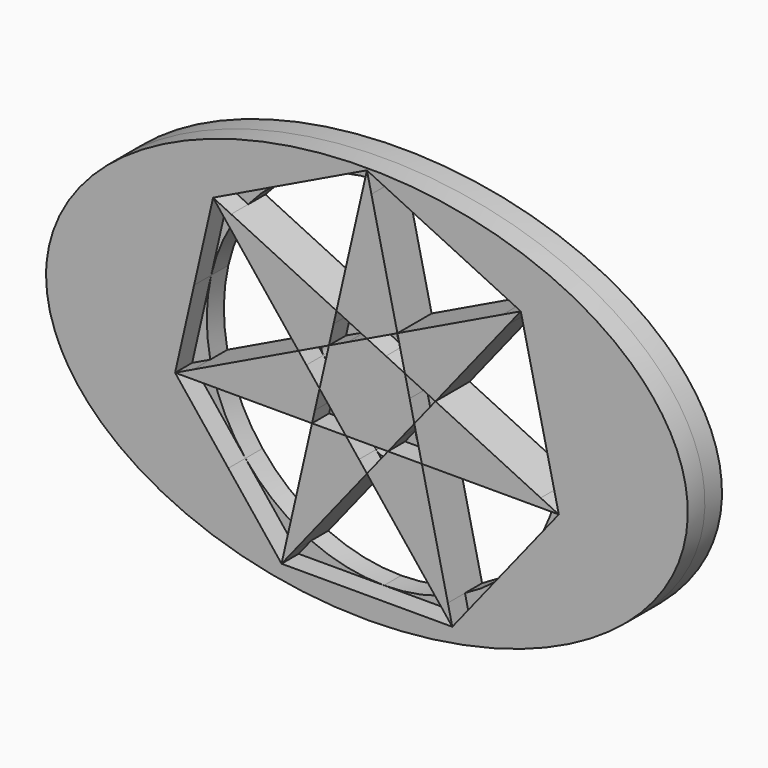
from build123d import *

# Parameters (mm, degrees)
F1_DEPTH = 5
F2_DEPTH = 5


# Not quite as in the source:
# - a feature names something its author has since deleted; it is built from what else it names


with BuildPart() as f1:
    # F0 (on Front) → F1 (new body, symmetric)
    with BuildSketch(Plane.XZ):
        with BuildLine():
            Line((-7.1231604273, 14.7913950385), (-31.742271471, 26.6473340548))
            ThreePointArc((-31.742271471, 26.6473340548), (-32.4026679799, 25.8402654428), (-33.0425496488, 25.0168367919))
            Line((-33.0425496488, 25.0168367919), (-16.0055961941, 3.653172885))
            Line((-16.0055961941, 3.653172885), (-13.3236535657, 4.944728384))
            Line((-13.3236535657, 4.944728384), (-8.8824357668, 7.0835061525))
            Line((-8.8824357668, 7.0835061525), (-7.7855455192, 11.8892963316))
            Line((-7.7855455192, 11.8892963316), (-7.1231604273, 14.7913950385))
        make_face()
        with BuildLine():
            Line((-31.742271471, 26.6473340548), (-35.9642481935, 28.6805308855))
            Line((-35.9642481935, 28.6805308855), (-33.0425496488, 25.0168367919))
            ThreePointArc((-33.0425496488, 25.0168367919), (-32.4026679799, 25.8402654428), (-31.742271471, 26.6473340548))
        make_face()
    extrude(amount=F1_DEPTH, both=True)


with BuildPart() as f1b:
    # F0 (on Front) → F1, piece 2 (new body, symmetric)
    with BuildSketch(Plane.XZ):
        with BuildLine():
            ThreePointArc((-40.6247072379, -8.2027661312), (-40.4054660769, -9.2222839618), (-40.1606433291, -10.235962962))
            Line((-40.1606433291, -10.235962962), (-12.8354915721, -10.235962962))
            Line((-12.8354915721, -10.235962962), (-12.1731064643, -7.3338641855))
            Line((-12.1731064643, -7.3338641855), (-11.0762162326, -2.528074076))
            Line((-11.0762162326, -2.528074076), (-14.1496343689, 1.3258703679))
            Line((-14.1496343689, 1.3258703679), (-16.0055961941, 3.653172885))
            Line((-16.0055961941, 3.653172885), (-40.6247072379, -8.2027661312))
        make_face()
        with BuildLine():
            Line((-40.6247072379, -8.2027661312), (-44.8466839604, -10.235962962))
            Line((-44.8466839604, -10.235962962), (-40.1606433291, -10.235962962))
            ThreePointArc((-40.1606433291, -10.235962962), (-40.4054660769, -9.2222839618), (-40.6247072379, -8.2027661312))
        make_face()
    extrude(amount=F1_DEPTH, both=True)


with BuildPart() as f1c:
    # F0 (on Front) → F1, piece 3 (new body, symmetric)
    with BuildSketch(Plane.XZ):
        with BuildLine():
            ThreePointArc((-18.9159098616, -36.8760161145), (-17.9821240968, -37.3402654428), (-17.0369534547, -37.7808738299))
            Line((-17.0369534547, -37.7808738299), (0, -16.417209923))
            Line((0, -16.417209923), (-1.85596184, -14.0899073875))
            Line((-1.85596184, -14.0899073875), (-4.9293799615, -10.235962962))
            Line((-4.9293799615, -10.235962962), (-9.8587599231, -10.235962962))
            Line((-9.8587599231, -10.235962962), (-12.8354915721, -10.235962962))
            Line((-12.8354915721, -10.235962962), (-18.9159098616, -36.8760161145))
        make_face()
        with BuildLine():
            Line((-18.9159098616, -36.8760161145), (-19.9586519994, -41.4445679235))
            Line((-19.9586519994, -41.4445679235), (-17.0369534547, -37.7808738299))
            ThreePointArc((-17.0369534547, -37.7808738299), (-17.9821240968, -37.3402654428), (-18.9159098616, -36.8760161145))
        make_face()
    extrude(amount=F1_DEPTH, both=True)


with BuildPart() as f1d:
    # F0 (on Front) → F1, piece 4 (new body, symmetric)
    with BuildSketch(Plane.XZ):
        with BuildLine():
            Line((0, -16.417209923), (17.0369534547, -37.7808738299))
            ThreePointArc((17.0369534547, -37.7808738299), (17.9821240968, -37.3402654428), (18.9159098616, -36.8760161145))
            Line((18.9159098616, -36.8760161145), (12.8354915721, -10.235962962))
            Line((12.8354915721, -10.235962962), (9.8587599151, -10.235962962))
            Line((9.8587599151, -10.235962962), (4.9293799615, -10.235962962))
            Line((4.9293799615, -10.235962962), (1.8559618555, -14.089907368))
            Line((1.8559618555, -14.089907368), (0, -16.417209923))
        make_face()
        with BuildLine():
            Line((17.0369534547, -37.7808738299), (19.9586519994, -41.4445679235))
            Line((19.9586519994, -41.4445679235), (18.9159098616, -36.8760161145))
            ThreePointArc((18.9159098616, -36.8760161145), (17.9821240968, -37.3402654428), (17.0369534547, -37.7808738299))
        make_face()
    extrude(amount=F1_DEPTH, both=True)


with BuildPart() as f1e:
    # F0 (on Front) → F1, piece 5 (new body, symmetric)
    with BuildSketch(Plane.XZ):
        with BuildLine():
            ThreePointArc((40.1606433291, -10.235962962), (40.4054660769, -9.2222839618), (40.6247072379, -8.2027661312))
            Line((40.6247072379, -8.2027661312), (16.0055961941, 3.653172885))
            Line((16.0055961941, 3.653172885), (14.1496343961, 1.3258704021))
            Line((14.1496343961, 1.3258704021), (11.0762162326, -2.528074076))
            Line((11.0762162326, -2.528074076), (12.1731064608, -7.3338641702))
            Line((12.1731064608, -7.3338641702), (12.8354915721, -10.235962962))
            Line((12.8354915721, -10.235962962), (40.1606433291, -10.235962962))
        make_face()
        with BuildLine():
            Line((40.1606433291, -10.235962962), (44.8466839604, -10.235962962))
            Line((44.8466839604, -10.235962962), (40.6247072379, -8.2027661312))
            ThreePointArc((40.6247072379, -8.2027661312), (40.4054660769, -9.2222839618), (40.1606433291, -10.235962962))
        make_face()
    extrude(amount=F1_DEPTH, both=True)


with BuildPart() as f1f:
    # F0 (on Front) → F1, piece 6 (new body, symmetric)
    with BuildSketch(Plane.XZ):
        with BuildLine():
            Line((16.0055961941, 3.653172885), (33.0425496488, 25.0168367919))
            ThreePointArc((33.0425496488, 25.0168367919), (32.4026679799, 25.8402654428), (31.742271471, 26.6473340548))
            Line((31.742271471, 26.6473340548), (7.1231604273, 14.7913950385))
            Line((7.1231604273, 14.7913950385), (7.7855455438, 11.8892962237))
            Line((7.7855455438, 11.8892962237), (8.8824357668, 7.0835061525))
            Line((8.8824357668, 7.0835061525), (13.3236536413, 4.9447283476))
            Line((13.3236536413, 4.9447283476), (16.0055961941, 3.653172885))
        make_face()
        with BuildLine():
            Line((33.0425496488, 25.0168367919), (35.9642481935, 28.6805308855))
            Line((35.9642481935, 28.6805308855), (31.742271471, 26.6473340548))
            ThreePointArc((31.742271471, 26.6473340548), (32.4026679799, 25.8402654428), (33.0425496488, 25.0168367919))
        make_face()
    extrude(amount=F1_DEPTH, both=True)


with BuildPart() as f1g:
    # F0 (on Front) → F1, piece 7 (new body, symmetric)
    with BuildSketch(Plane.XZ):
        with BuildLine():
            Line((7.1231604273, 14.7913950385), (1.0427421378, 41.431448191))
            ThreePointArc((1.0427421378, 41.431448191), (0, 41.4445679235), (-1.0427421378, 41.431448191))
            Line((-1.0427421378, 41.431448191), (-7.1231604273, 14.7913950385))
            Line((-7.1231604273, 14.7913950385), (-4.4412178209, 13.4998395501))
            Line((-4.4412178209, 13.4998395501), (0, 11.361061771))
            Line((0, 11.361061771), (4.4412179301, 13.4998396027))
            Line((4.4412179301, 13.4998396027), (7.1231604273, 14.7913950385))
        make_face()
        with BuildLine():
            Line((1.0427421378, 41.431448191), (0, 46))
            Line((0, 46), (-1.0427421378, 41.431448191))
            ThreePointArc((-1.0427421378, 41.431448191), (0, 41.4445679235), (1.0427421378, 41.431448191))
        make_face()
    extrude(amount=F1_DEPTH, both=True)


with BuildPart() as f1h:
    # F0 (on Front) → F1, piece 8 (new body, symmetric)
    with BuildSketch(Plane.XZ):
        with BuildLine():
            add(Edge.make_bspline(
                [(-75, 0), (-75, -80.540362552), (37.5, -40.270181276), (150, 0), (37.5, 40.270181276), (-75, 80.540362552), (-75, 0)],
                knots=[0, 0, 0, 2.0943951024, 2.0943951024, 4.1887902048, 4.1887902048, 6.2831853072, 6.2831853072, 6.2831853072], degree=2, weights=[1, 0.5, 1, 0.5, 1, 0.5, 1]))
        make_face()
        with BuildLine():
            ThreePointArc((35.9642481935, 28.6805308855), (43.4186331942, 15.1928368499), (46, 0))
            ThreePointArc((46, 0), (45.7107616551, -5.1503659008), (44.8466839604, -10.235962962))
            ThreePointArc((44.8466839604, -10.235962962), (35.9642481935, -28.6805308855), (19.9586519994, -41.4445679235))
            ThreePointArc((19.9586519994, -41.4445679235), (0, -46), (-19.9586519994, -41.4445679235))
            ThreePointArc((-19.9586519994, -41.4445679235), (-35.9642481935, -28.6805308855), (-44.8466839604, -10.235962962))
            ThreePointArc((-44.8466839604, -10.235962962), (-44.8466839604, 10.235962962), (-35.9642481935, 28.6805308855))
            ThreePointArc((-35.9642481935, 28.6805308855), (-19.9586519994, 41.4445679235), (0, 46))
            ThreePointArc((0, 46), (19.9586519994, 41.4445679235), (35.9642481935, 28.6805308855))
        make_face(mode=Mode.SUBTRACT)
        with BuildLine():
            ThreePointArc((-19.9586519994, -41.4445679235), (0, -46), (19.9586519994, -41.4445679235))
            Line((19.9586519994, -41.4445679235), (-1.551e-07, -41.4445679235))
            Line((-1.551e-07, -41.4445679235), (-19.9586519994, -41.4445679235))
        make_face()
        with BuildLine():
            ThreePointArc((-44.8466839604, -10.235962962), (-35.9642481935, -28.6805308855), (-19.9586519994, -41.4445679235))
            Line((-19.9586519994, -41.4445679235), (-32.4026679565, -25.840265472))
            Line((-32.4026679565, -25.840265472), (-44.8466839604, -10.235962962))
        make_face()
        with BuildLine():
            Line((-40.405466174, 9.2222835364), (-35.9642481935, 28.6805308855))
            ThreePointArc((-35.9642481935, 28.6805308855), (-44.8466839604, 10.235962962), (-44.8466839604, -10.235962962))
            Line((-44.8466839604, -10.235962962), (-40.405466174, 9.2222835364))
        make_face()
        with BuildLine():
            Line((-17.9821241425, 37.3402654207), (0, 46))
            ThreePointArc((0, 46), (-19.9586519994, 41.4445679235), (-35.9642481935, 28.6805308855))
            Line((-35.9642481935, 28.6805308855), (-17.9821241425, 37.3402654207))
        make_face()
        with BuildLine():
            Line((17.982124206, 37.3402653901), (35.9642481935, 28.6805308855))
            ThreePointArc((35.9642481935, 28.6805308855), (19.9586519994, 41.4445679235), (0, 46))
            Line((0, 46), (17.982124206, 37.3402653901))
        make_face()
        with BuildLine():
            ThreePointArc((44.8466839604, -10.235962962), (45.7107616551, -5.1503659008), (46, 0))
            ThreePointArc((46, 0), (43.4186331942, 15.1928368499), (35.9642481935, 28.6805308855))
            Line((35.9642481935, 28.6805308855), (40.4054662225, 9.2222833239))
            Line((40.4054662225, 9.2222833239), (44.8466839604, -10.235962962))
        make_face()
        with BuildLine():
            ThreePointArc((19.9586519994, -41.4445679235), (35.9642481935, -28.6805308855), (44.8466839604, -10.235962962))
            Line((44.8466839604, -10.235962962), (32.402668315, -25.8402650225))
            Line((32.402668315, -25.8402650225), (19.9586519994, -41.4445679235))
        make_face()
    extrude(amount=F1_DEPTH, both=True)


with BuildPart() as f1i:
    # F0 (on Front) → F1, piece 9 (new body, symmetric)
    with BuildSketch(Plane.XZ):
        Polygon((9.9793259997, 2.2777160382), (8.8824357668, 7.0835061525), (4.4412178834, 9.2222839618), (0, 11.361061771), (-4.4412178834, 9.2222839618), (-8.8824357668, 7.0835061525), (-9.9793259997, 2.2777160382), (-11.0762162326, -2.528074076), (-8.0027980971, -6.382018519), (-4.9293799615, -10.235962962), (0, -10.235962962), (4.9293799615, -10.235962962), (8.0027980971, -6.382018519), (11.0762162326, -2.528074076), align=None)
    extrude(amount=F1_DEPTH, both=True)


with BuildPart() as f2:
    # F0 (on Front) → F2 (new body)
    with BuildSketch(Plane.XZ):
        with BuildLine():
            Line((-33.0425496488, 25.0168367919), (-35.9642481935, 28.6805308855))
            Line((-35.9642481935, 28.6805308855), (-40.405466174, 9.2222835364))
            ThreePointArc((-40.405466174, 9.2222835364), (-37.563542634, 17.5109244517), (-33.0425496488, 25.0168367919))
        make_face()
    extrude(amount=-F2_DEPTH)


with BuildPart() as f2b:
    # F0 (on Front) → F2, piece 2 (new body)
    with BuildSketch(Plane.XZ):
        with BuildLine():
            Line((-17.9821241425, 37.3402654207), (-35.9642481935, 28.6805308855))
            Line((-35.9642481935, 28.6805308855), (-31.742271471, 26.6473340548))
            ThreePointArc((-31.742271471, 26.6473340548), (-25.430563798, 32.7251987814), (-17.9821241425, 37.3402654207))
        make_face()
    extrude(amount=-F2_DEPTH)


with BuildPart() as f2c:
    # F0 (on Front) → F2, piece 3 (new body)
    with BuildSketch(Plane.XZ):
        with BuildLine():
            Line((-1.0427421378, 41.431448191), (0, 46))
            Line((0, 46), (-17.9821241425, 37.3402654207))
            ThreePointArc((-17.9821241425, 37.3402654207), (-9.7298935432, 40.2862430863), (-1.0427421378, 41.431448191))
        make_face()
    extrude(amount=-F2_DEPTH)


with BuildPart() as f2d:
    # F0 (on Front) → F2, piece 4 (new body)
    with BuildSketch(Plane.XZ):
        with BuildLine():
            Line((17.982124206, 37.3402653901), (0, 46))
            Line((0, 46), (1.0427421378, 41.431448191))
            ThreePointArc((1.0427421378, 41.431448191), (9.7298935774, 40.286243078), (17.982124206, 37.3402653901))
        make_face()
    extrude(amount=-F2_DEPTH)


with BuildPart() as f2e:
    # F0 (on Front) → F2, piece 5 (new body)
    with BuildSketch(Plane.XZ):
        with BuildLine():
            Line((31.742271471, 26.6473340548), (35.9642481935, 28.6805308855))
            Line((35.9642481935, 28.6805308855), (17.982124206, 37.3402653901))
            ThreePointArc((17.982124206, 37.3402653901), (25.4305638258, 32.7251987598), (31.742271471, 26.6473340548))
        make_face()
    extrude(amount=-F2_DEPTH)


with BuildPart() as f2f:
    # F0 (on Front) → F2, piece 6 (new body)
    with BuildSketch(Plane.XZ):
        with BuildLine():
            Line((40.4054662225, 9.2222833239), (35.9642481935, 28.6805308855))
            Line((35.9642481935, 28.6805308855), (33.0425496488, 25.0168367919))
            ThreePointArc((33.0425496488, 25.0168367919), (37.56354268, 17.5109243529), (40.4054662225, 9.2222833239))
        make_face()
    extrude(amount=-F2_DEPTH)


with BuildPart() as f2g:
    # F0 (on Front) → F2, piece 7 (new body)
    with BuildSketch(Plane.XZ):
        with BuildLine():
            Line((40.6247072379, -8.2027661312), (44.8466839604, -10.235962962))
            Line((44.8466839604, -10.235962962), (40.4054662225, 9.2222833239))
            ThreePointArc((40.4054662225, 9.2222833239), (41.183973216, 4.6403190098), (41.4445679235, 0))
            ThreePointArc((41.4445679235, 0), (41.2390933997, -4.1218182804), (40.6247072379, -8.2027661312))
        make_face()
    extrude(amount=-F2_DEPTH)


with BuildPart() as f2h:
    # F0 (on Front) → F2, piece 8 (new body)
    with BuildSketch(Plane.XZ):
        with BuildLine():
            Line((32.402668315, -25.8402650225), (44.8466839604, -10.235962962))
            Line((44.8466839604, -10.235962962), (40.1606433291, -10.235962962))
            ThreePointArc((40.1606433291, -10.235962962), (37.1110779942, -18.4504769716), (32.402668315, -25.8402650225))
        make_face()
    extrude(amount=-F2_DEPTH)


with BuildPart() as f2i:
    # F0 (on Front) → F2, piece 9 (new body)
    with BuildSketch(Plane.XZ):
        with BuildLine():
            Line((18.9159098616, -36.8760161145), (19.9586519994, -41.4445679235))
            Line((19.9586519994, -41.4445679235), (32.402668315, -25.8402650225))
            ThreePointArc((32.402668315, -25.8402650225), (26.245877144, -32.0750080796), (18.9159098616, -36.8760161145))
        make_face()
    extrude(amount=-F2_DEPTH)


with BuildPart() as f2j:
    # F0 (on Front) → F2, piece 10 (new body)
    with BuildSketch(Plane.XZ):
        with BuildLine():
            Line((-1.551e-07, -41.4445679235), (19.9586519994, -41.4445679235))
            Line((19.9586519994, -41.4445679235), (17.0369534547, -37.7808738299))
            ThreePointArc((17.0369534547, -37.7808738299), (8.7132145639, -40.5182934282), (-1.551e-07, -41.4445679235))
        make_face()
    extrude(amount=-F2_DEPTH)


with BuildPart() as f2k:
    # F0 (on Front) → F2, piece 11 (new body)
    with BuildSketch(Plane.XZ):
        with BuildLine():
            Line((-17.0369534547, -37.7808738299), (-19.9586519994, -41.4445679235))
            Line((-19.9586519994, -41.4445679235), (-1.551e-07, -41.4445679235))
            ThreePointArc((-1.551e-07, -41.4445679235), (-8.7132147155, -40.5182933956), (-17.0369534547, -37.7808738299))
        make_face()
    extrude(amount=-F2_DEPTH)


with BuildPart() as f2l:
    # F0 (on Front) → F2, piece 12 (new body)
    with BuildSketch(Plane.XZ):
        with BuildLine():
            Line((-32.4026679565, -25.840265472), (-19.9586519994, -41.4445679235))
            Line((-19.9586519994, -41.4445679235), (-18.9159098616, -36.8760161145))
            ThreePointArc((-18.9159098616, -36.8760161145), (-26.2458769215, -32.0750082617), (-32.4026679565, -25.840265472))
        make_face()
    extrude(amount=-F2_DEPTH)


with BuildPart() as f2m:
    # F0 (on Front) → F2, piece 13 (new body)
    with BuildSketch(Plane.XZ):
        with BuildLine():
            Line((-40.1606433291, -10.235962962), (-44.8466839604, -10.235962962))
            Line((-44.8466839604, -10.235962962), (-32.4026679565, -25.840265472))
            ThreePointArc((-32.4026679565, -25.840265472), (-37.1110778662, -18.450477229), (-40.1606433291, -10.235962962))
        make_face()
    extrude(amount=-F2_DEPTH)


with BuildPart() as f2n:
    # F0 (on Front) → F2, piece 14 (new body)
    with BuildSketch(Plane.XZ):
        with BuildLine():
            Line((-40.405466174, 9.2222835364), (-44.8466839604, -10.235962962))
            Line((-44.8466839604, -10.235962962), (-40.6247072379, -8.2027661312))
            ThreePointArc((-40.6247072379, -8.2027661312), (-41.4412878633, 0.5214121171), (-40.405466174, 9.2222835364))
        make_face()
    extrude(amount=-F2_DEPTH)


with BuildPart() as f2o:
    # F0 (on Front) → F2, piece 15 (new body)
    with BuildSketch(Plane.XZ):
        with BuildLine():
            ThreePointArc((-4.4412178834, 9.2222839618), (-6.9512791847, 9.5050999657), (-7.7855455192, 11.8892963316))
            Line((-7.7855455192, 11.8892963316), (-8.8824357668, 7.0835061525))
            Line((-8.8824357668, 7.0835061525), (-4.4412178834, 9.2222839618))
        make_face()
    extrude(amount=-F2_DEPTH)


with BuildPart() as f2p:
    # F0 (on Front) → F2, piece 16 (new body)
    with BuildSketch(Plane.XZ):
        with BuildLine():
            Line((-6.5011800998, 13.4998395803), (-7.1231604273, 14.7913950385))
            Line((-7.1231604273, 14.7913950385), (-7.7855455192, 11.8892963316))
            ThreePointArc((-7.7855455192, 11.8892963316), (-7.3271607969, 12.8411419641), (-6.5011800998, 13.4998395803))
        make_face()
        with BuildLine():
            Line((-4.4412178209, 13.4998395501), (-7.1231604273, 14.7913950385))
            Line((-7.1231604273, 14.7913950385), (-6.5011800998, 13.4998395803))
            ThreePointArc((-6.5011800998, 13.4998395803), (-5.4711989569, 13.7349260469), (-4.4412178209, 13.4998395501))
        make_face()
    extrude(amount=-F2_DEPTH)


with BuildPart() as f2q:
    # F0 (on Front) → F2, piece 17 (new body)
    with BuildSketch(Plane.XZ):
        with BuildLine():
            Line((0, 11.361061771), (-4.4412178209, 13.4998395501))
            ThreePointArc((-4.4412178209, 13.4998395501), (-3.461190645, 12.6240336817), (-3.0973347157, 11.361061771))
            ThreePointArc((-3.0973347157, 11.361061771), (-3.4611906635, 10.0980898309), (-4.4412178834, 9.2222839618))
            Line((-4.4412178834, 9.2222839618), (0, 11.361061771))
        make_face()
    extrude(amount=-F2_DEPTH)


with BuildPart() as f2r:
    # F0 (on Front) → F2, piece 18 (new body)
    with BuildSketch(Plane.XZ):
        with BuildLine():
            Line((7.7855455438, 11.8892962237), (7.1231604273, 14.7913950385))
            Line((7.1231604273, 14.7913950385), (6.5011800998, 13.4998395803))
            ThreePointArc((6.5011800998, 13.4998395803), (7.3271608314, 12.8411419208), (7.7855455438, 11.8892962237))
        make_face()
        with BuildLine():
            Line((6.5011800998, 13.4998395803), (7.1231604273, 14.7913950385))
            Line((7.1231604273, 14.7913950385), (4.4412179301, 13.4998396027))
            ThreePointArc((4.4412179301, 13.4998396027), (5.4711990175, 13.7349260469), (6.5011800998, 13.4998395803))
        make_face()
    extrude(amount=-F2_DEPTH)


with BuildPart() as f2s:
    # F0 (on Front) → F2, piece 19 (new body)
    with BuildSketch(Plane.XZ):
        with BuildLine():
            Line((8.8824357668, 7.0835061525), (7.7855455438, 11.8892962237))
            ThreePointArc((7.7855455438, 11.8892962237), (7.8301369097, 11.626850219), (7.8450632676, 11.361061771))
            ThreePointArc((7.8450632676, 11.361061771), (6.7341709317, 9.3510534429), (4.4412178834, 9.2222839618))
            Line((4.4412178834, 9.2222839618), (8.8824357668, 7.0835061525))
        make_face()
    extrude(amount=-F2_DEPTH)


with BuildPart() as f2t:
    # F0 (on Front) → F2, piece 20 (new body)
    with BuildSketch(Plane.XZ):
        with BuildLine():
            ThreePointArc((9.9793259997, 2.2777160382), (10.8135923711, 4.6619123569), (13.3236536413, 4.9447283476))
            Line((13.3236536413, 4.9447283476), (8.8824357668, 7.0835061525))
            Line((8.8824357668, 7.0835061525), (9.9793259997, 2.2777160382))
        make_face()
    extrude(amount=-F2_DEPTH)


with BuildPart() as f2u:
    # F0 (on Front) → F2, piece 21 (new body)
    with BuildSketch(Plane.XZ):
        with BuildLine():
            ThreePointArc((4.4412178834, 9.2222839618), (3.0973347157, 11.3610617969), (4.4412179301, 13.4998396027))
            Line((4.4412179301, 13.4998396027), (0, 11.361061771))
            Line((0, 11.361061771), (4.4412178834, 9.2222839618))
        make_face()
    extrude(amount=-F2_DEPTH)


with BuildPart() as f2v:
    # F0 (on Front) → F2, piece 22 (new body)
    with BuildSketch(Plane.XZ):
        with BuildLine():
            Line((14.6080190844, 3.3341850298), (16.0055961941, 3.653172885))
            Line((16.0055961941, 3.653172885), (13.3236536413, 4.9447283476))
            ThreePointArc((13.3236536413, 4.9447283476), (14.149634365, 4.286030705), (14.6080190844, 3.3341850298))
        make_face()
        with BuildLine():
            Line((14.1496343961, 1.3258704021), (16.0055961941, 3.653172885))
            Line((16.0055961941, 3.653172885), (14.6080190844, 3.3341850298))
            ThreePointArc((14.6080190844, 3.3341850298), (14.6526104577, 3.071739004), (14.667536818, 2.805950534))
            ThreePointArc((14.667536818, 2.805950534), (14.5343234679, 2.021912889), (14.1496343961, 1.3258704021))
        make_face()
    extrude(amount=-F2_DEPTH)


with BuildPart() as f2w:
    # F0 (on Front) → F2, piece 23 (new body)
    with BuildSketch(Plane.XZ):
        with BuildLine():
            Line((11.0762162326, -2.528074076), (14.1496343961, 1.3258704021))
            ThreePointArc((14.1496343961, 1.3258704021), (11.7654380682, 0.4916039867), (9.9793259997, 2.2777160382))
            Line((9.9793259997, 2.2777160382), (11.0762162326, -2.528074076))
        make_face()
    extrude(amount=-F2_DEPTH)


with BuildPart() as f2x:
    # F0 (on Front) → F2, piece 24 (new body)
    with BuildSketch(Plane.XZ):
        with BuildLine():
            ThreePointArc((8.0027980971, -6.382018519), (10.3869944088, -5.5477521414), (12.1731064608, -7.3338641702))
            Line((12.1731064608, -7.3338641702), (11.0762162326, -2.528074076))
            Line((11.0762162326, -2.528074076), (8.0027980971, -6.382018519))
        make_face()
    extrude(amount=-F2_DEPTH)


with BuildPart() as f2y:
    # F0 (on Front) → F2, piece 25 (new body)
    with BuildSketch(Plane.XZ):
        with BuildLine():
            Line((11.7147217491, -9.3421788531), (12.8354915721, -10.235962962))
            Line((12.8354915721, -10.235962962), (12.1731064608, -7.3338641702))
            ThreePointArc((12.1731064608, -7.3338641702), (12.2176978376, -7.5963102058), (12.232624199, -7.8620986861))
            ThreePointArc((12.232624199, -7.8620986861), (12.0994108416, -8.6461363523), (11.7147217491, -9.3421788531))
        make_face()
        with BuildLine():
            Line((9.8587599151, -10.235962962), (12.8354915721, -10.235962962))
            Line((12.8354915721, -10.235962962), (11.7147217491, -9.3421788531))
            ThreePointArc((11.7147217491, -9.3421788531), (10.8887410277, -10.000876497), (9.8587599151, -10.235962962))
        make_face()
    extrude(amount=-F2_DEPTH)


with BuildPart() as f2z:
    # F0 (on Front) → F2, piece 26 (new body)
    with BuildSketch(Plane.XZ):
        with BuildLine():
            Line((4.9293799615, -10.235962962), (9.8587599151, -10.235962962))
            ThreePointArc((9.8587599151, -10.235962962), (7.7199821121, -8.8920797906), (8.0027980971, -6.382018519))
            Line((8.0027980971, -6.382018519), (4.9293799615, -10.235962962))
        make_face()
    extrude(amount=-F2_DEPTH)


with BuildPart() as f2ba:
    # F0 (on Front) → F2, piece 27 (new body)
    with BuildSketch(Plane.XZ):
        with BuildLine():
            ThreePointArc((2.3738642759, -12.6098272379), (2.2406509263, -13.3938648819), (1.8559618555, -14.089907368))
            Line((1.8559618555, -14.089907368), (4.9293799615, -10.235962962))
            Line((4.9293799615, -10.235962962), (0, -10.235962962))
            ThreePointArc((0, -10.235962962), (1.6785755271, -10.9312517108), (2.3738642759, -12.6098272379))
        make_face()
    extrude(amount=-F2_DEPTH)


with BuildPart() as f2bb:
    # F0 (on Front) → F2, piece 28 (new body)
    with BuildSketch(Plane.XZ):
        with BuildLine():
            Line((-4.9293799615, -10.235962962), (-1.85596184, -14.0899073875))
            ThreePointArc((-1.85596184, -14.0899073875), (-2.1387778044, -11.5798461197), (0, -10.235962962))
            Line((0, -10.235962962), (-4.9293799615, -10.235962962))
        make_face()
    extrude(amount=-F2_DEPTH)


with BuildPart() as f2bc:
    # F0 (on Front) → F2, piece 29 (new body)
    with BuildSketch(Plane.XZ):
        with BuildLine():
            Line((-1.85596184, -14.0899073875), (0, -16.417209923))
            Line((0, -16.417209923), (0, -14.9836915139))
            ThreePointArc((0, -14.9836915139), (-1.0299811183, -14.7486050423), (-1.85596184, -14.0899073875))
        make_face()
        with BuildLine():
            Line((0, -14.9836915139), (0, -16.417209923))
            Line((0, -16.417209923), (1.8559618555, -14.089907368))
            ThreePointArc((1.8559618555, -14.089907368), (1.0299811295, -14.7486050369), (0, -14.9836915139))
        make_face()
    extrude(amount=-F2_DEPTH)


with BuildPart() as f2bd:
    # F0 (on Front) → F2, piece 30 (new body)
    with BuildSketch(Plane.XZ):
        with BuildLine():
            ThreePointArc((-7.4848956472, -7.8620986861), (-8.180184396, -9.5406742132), (-9.8587599231, -10.235962962))
            Line((-9.8587599231, -10.235962962), (-4.9293799615, -10.235962962))
            Line((-4.9293799615, -10.235962962), (-8.0027980971, -6.382018519))
            ThreePointArc((-8.0027980971, -6.382018519), (-7.6181090046, -7.0780610198), (-7.4848956472, -7.8620986861))
        make_face()
    extrude(amount=-F2_DEPTH)


with BuildPart() as f2be:
    # F0 (on Front) → F2, piece 31 (new body)
    with BuildSketch(Plane.XZ):
        with BuildLine():
            Line((-11.0762162326, -2.528074076), (-12.1731064643, -7.3338641855))
            ThreePointArc((-12.1731064643, -7.3338641855), (-10.3869944165, -5.5477521432), (-8.0027980971, -6.382018519))
            Line((-8.0027980971, -6.382018519), (-11.0762162326, -2.528074076))
        make_face()
    extrude(amount=-F2_DEPTH)


with BuildPart() as f2bf:
    # F0 (on Front) → F2, piece 32 (new body)
    with BuildSketch(Plane.XZ):
        with BuildLine():
            Line((-12.1731064643, -7.3338641855), (-12.8354915721, -10.235962962))
            Line((-12.8354915721, -10.235962962), (-11.7147217491, -9.3421788531))
            ThreePointArc((-11.7147217491, -9.3421788531), (-12.173106466, -8.3903331794), (-12.1731064643, -7.3338641855))
        make_face()
        with BuildLine():
            Line((-11.7147217491, -9.3421788531), (-12.8354915721, -10.235962962))
            Line((-12.8354915721, -10.235962962), (-9.8587599231, -10.235962962))
            ThreePointArc((-9.8587599231, -10.235962962), (-10.8887410313, -10.0008764953), (-11.7147217491, -9.3421788531))
        make_face()
    extrude(amount=-F2_DEPTH)


with BuildPart() as f2bg:
    # F0 (on Front) → F2, piece 33 (new body)
    with BuildSketch(Plane.XZ):
        with BuildLine():
            ThreePointArc((-9.9793259997, 2.2777160382), (-11.7654380469, 0.4916039915), (-14.1496343689, 1.3258703679))
            Line((-14.1496343689, 1.3258703679), (-11.0762162326, -2.528074076))
            Line((-11.0762162326, -2.528074076), (-9.9793259997, 2.2777160382))
        make_face()
    extrude(amount=-F2_DEPTH)


with BuildPart() as f2bh:
    # F0 (on Front) → F2, piece 34 (new body)
    with BuildSketch(Plane.XZ):
        with BuildLine():
            Line((-8.8824357668, 7.0835061525), (-13.3236535657, 4.944728384))
            ThreePointArc((-13.3236535657, 4.944728384), (-11.0307005622, 4.8159588372), (-9.9198082661, 2.805950534))
            ThreePointArc((-9.9198082661, 2.805950534), (-9.9347346264, 2.540162064), (-9.9793259997, 2.2777160382))
            Line((-9.9793259997, 2.2777160382), (-8.8824357668, 7.0835061525))
        make_face()
    extrude(amount=-F2_DEPTH)


with BuildPart() as f2bi:
    # F0 (on Front) → F2, piece 35 (new body)
    with BuildSketch(Plane.XZ):
        with BuildLine():
            Line((-13.3236535657, 4.944728384), (-16.0055961941, 3.653172885))
            Line((-16.0055961941, 3.653172885), (-14.6080190844, 3.3341850298))
            ThreePointArc((-14.6080190844, 3.3341850298), (-14.1496343388, 4.2860307378), (-13.3236535657, 4.944728384))
        make_face()
        with BuildLine():
            Line((-14.6080190844, 3.3341850298), (-16.0055961941, 3.653172885))
            Line((-16.0055961941, 3.653172885), (-14.1496343689, 1.3258703679))
            ThreePointArc((-14.1496343689, 1.3258703679), (-14.6080190845, 2.2777160389), (-14.6080190844, 3.3341850298))
        make_face()
    extrude(amount=-F2_DEPTH)


solid = Compound([f1.part, f1b.part, f1c.part, f1d.part, f1e.part, f1f.part, f1g.part, f1h.part, f1i.part, f2.part, f2b.part, f2c.part, f2d.part, f2e.part, f2f.part, f2g.part, f2h.part, f2i.part, f2j.part, f2k.part, f2l.part, f2m.part, f2n.part, f2o.part, f2p.part, f2q.part, f2r.part, f2s.part, f2t.part, f2u.part, f2v.part, f2w.part, f2x.part, f2y.part, f2z.part, f2ba.part, f2bb.part, f2bc.part, f2bd.part, f2be.part, f2bf.part, f2bg.part, f2bh.part, f2bi.part])
